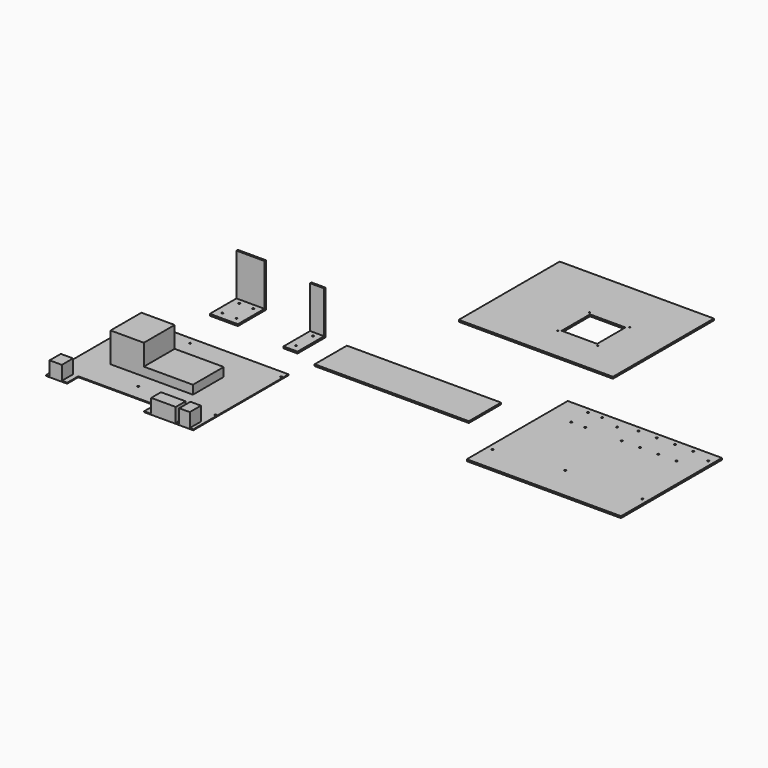
from build123d import *

# Parameters (mm, degrees)
F1_DEPTH  = 1.5875
F2_W      = 22.225
F2_H      = 25.4
F3_DEPTH  = 22.225
F2_W_2    = 44.45
F2_H_2    = 22.225
F4_DEPTH  = 25.4
F5_W      = 88.9
F5_H      = 69.85
F6_DEPTH  = 15.875
F7_W      = 60.325
F7_H      = 69.85
F8_DEPTH  = 53.975
F10_DEPTH = 3.175
F11_W     = 50.8
F11_H     = 63.5
F12_DEPTH = 3.175
F11_W_2   = 25.4
F13_W     = 50.8
F13_H     = 3.175
F14_DEPTH = 76.2
F16_D     = 3.175
F18_D     = 3.175
F20_D     = 3.175
F21_W     = 25.4
F21_H     = 3.175
F22_DEPTH = 76.2
F24_D     = 3.175
F25_W     = 279.4
F25_H     = 73.025
F26_DEPTH = 2.9972
F27_W     = 279.4
F27_H     = 228.6
F27_W_2   = 79.502
F27_H_2   = 79.502
F27_W_3   = 64.262
F27_H_3   = 64.262
F28_DEPTH = 3.175
F30_D     = 2.0066


# Not quite as in the source:
# - a feature names something its author has since deleted; it is built from what else it names


with BuildPart() as f1:
    # F0 (on Top) → F1 (new body)
    with BuildSketch(Plane.XY):
        Polygon((133.9049825728, 35.3928071586), (-132.7950174272, 35.3928071586), (-132.7950174272, -180.5071928414), (-94.6950174272, -180.5071928414), (-94.6950174272, -155.1071928414), (45.0049825728, -155.1071928414), (45.0049825728, -180.5071928414), (133.9049825728, -180.5071928414), align=None)
    extrude(amount=F1_DEPTH)

    # F2 (on face) → F3 (join)
    with BuildSketch(Plane.XY.offset(1.5875)):
        with Locations((-115.3325174272, -167.8071928414)):
            Rectangle(F2_W, F2_H)
    extrude(amount=F3_DEPTH)

    # F2 (on face) → F4 (join)
    with BuildSketch(Plane.XY.offset(1.5875)):
        with Locations((-115.3325174272, -167.8071928414)):
            Rectangle(F2_W, F2_H)
        with Locations((79.9299825728, -169.3946928414)):
            Rectangle(F2_W_2, F2_H_2)
        Polygon((127.5549825728, -155.1073775974), (108.4081034214, -155.1073775974), (108.5049825728, -180.5071928414), (127.5549825728, -180.5071928414), align=None)
    extrude(amount=F4_DEPTH)

    # F5 (on face) → F6 (join)
    with BuildSketch(Plane.XY.offset(1.5875)):
        with Locations((22.7799825728, -63.0321928414)):
            Rectangle(F5_W, F5_H)
    extrude(amount=F6_DEPTH)

    # F7 (on face) → F8 (join)
    with BuildSketch(Plane.XY.offset(1.5875)):
        with Locations((-51.8325174272, -63.0321928414)):
            Rectangle(F7_W, F7_H)
    extrude(amount=F8_DEPTH)

    # F16 (through all)
    with Locations(Plane.XY.offset(1.5875)):
        with Locations((-129.6200174272, -140.8196928414), (-8.9700174272, -126.5321928414), (130.7299825728, -126.5321928414), (130.7299825728, 22.6928071586), (-34.3700174272, 22.6928071586)):
            Hole(F16_D / 2)


with BuildPart() as f10:
    # F9 (on Top) → F10 (new body)
    with BuildSketch(Plane.XY):
        Polygon((774.6669458253, 216.0189813188), (495.2669458253, 216.0189813188), (495.2669458253, -12.5810186812), (539.7169458253, -12.5810186812), (692.1169458253, -12.5810186812), (774.6669458253, -12.5810186812), align=None)
    extrude(amount=F10_DEPTH)

    # F18 (through all)
    with Locations(Plane.XY.offset(3.175)):
        with Locations((504.7919458253, 33.4437813188), (625.4419458253, 47.7439813188), (765.1419458253, 47.7439813188), (765.1419458253, 196.9689813188), (600.0419458253, 196.9689813188), (565.1169458253, 168.3939813188), (565.1169458253, 206.4939813188), (539.7169458253, 206.4939813188), (539.7169458253, 168.3939813188), (631.1569458253, 206.4939813188), (664.1769458253, 206.4939813188), (697.1969458253, 206.4939813188), (730.2169458253, 206.4939813188), (664.1769458253, 168.3939813188), (697.1969458253, 168.3939813188), (730.2169458253, 168.3939813188), (631.1569458253, 168.3939813188)):
            Hole(F18_D / 2)


with BuildPart() as f12:
    # F11 (on Top) → F12 (new body)
    with BuildSketch(Plane.XY):
        with Locations((-41.6685035452, 139.9601322776)):
            Rectangle(F11_W, F11_H)
    extrude(amount=F12_DEPTH)

    # F13 (on face) → F14 (join)
    with BuildSketch(Plane.XY.offset(3.175)):
        with Locations((-41.6685035452, 170.1226322776)):
            Rectangle(F13_W, F13_H)
    extrude(amount=F14_DEPTH)

    # F20 (through all)
    with Locations(Plane.XY.offset(3.175)):
        with Locations((-54.3685035452, 120.9101322776), (-28.9685035452, 120.9101322776), (-28.825070553, 159.0101322776), (-54.4048526267, 159.0101322776)):
            Hole(F20_D / 2)


with BuildPart() as f12b:
    # F11 (on Top) → F12, piece 2 (new body)
    with BuildSketch(Plane.XY):
        with Locations((89.4274200916, 127.0945136547)):
            Rectangle(F11_W_2, F11_H)
    extrude(amount=F12_DEPTH)

    # F21 (on face) → F22 (join)
    with BuildSketch(Plane.XY.offset(3.175)):
        with Locations((89.4274200916, 157.2570136547)):
            Rectangle(F21_W, F21_H)
    extrude(amount=F22_DEPTH)

    # F24 (through all)
    with Locations(Plane.XY.offset(3.175)):
        with Locations((89.4274200916, 146.1445136547), (89.4274200916, 108.0445136547)):
            Hole(F24_D / 2)


with BuildPart() as f26:
    # F25 (on Top) → F26 (new body)
    with BuildSketch(Plane.XY):
        with Locations((284.80287323, 116.9579862564)):
            Rectangle(F25_W, F25_H)
    extrude(amount=F26_DEPTH)


with BuildPart() as f28:
    # F27 (on Top) → F28 (new body)
    with BuildSketch(Plane.XY):
        with Locations((359.1902479529, 428.1840278369)):
            Rectangle(F27_W, F27_H)
        with Locations((386.2412479529, 410.7850278369)):
            Rectangle(F27_W_2, F27_H_2, mode=Mode.SUBTRACT)
        with Locations((386.2412479529, 410.7850278369)):
            Rectangle(F27_W_2, F27_H_2)
        with Locations((386.2412479529, 410.7850278369)):
            Rectangle(F27_W_3, F27_H_3, mode=Mode.SUBTRACT)
    extrude(amount=F28_DEPTH)

    # F30 (through all)
    with Locations(Plane.XY.offset(3.175)):
        with Locations((349.9954479529, 447.0308278369), (422.4870479529, 447.0308278369), (422.4870479529, 374.9376833439), (349.9954479529, 374.9376833439)):
            Hole(F30_D / 2)


solid = Compound([f1.part, f10.part, f12.part, f12b.part, f26.part, f28.part])
